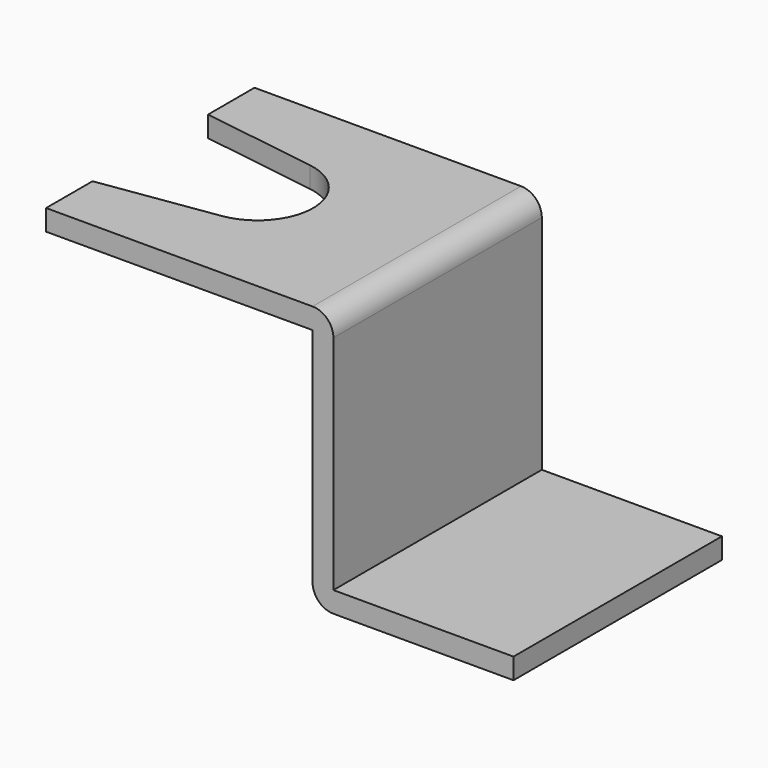
from build123d import *

# Parameters (mm, degrees)
F1_DEPTH = 25
F2_R     = 5.3407247833
F3_DEPTH = 25.3101193046
F5_DEPTH = 106
F6_DEPTH = 25.3101193046


# Not quite as in the source:
# - an extrude ends at something that could not be found from the text; its depth is read off the source's solid


with BuildPart() as f1:
    # F0 (on Front) → F1 (new body)
    with BuildSketch(Plane.XZ):
        with BuildLine():
            Line((-2, 0), (-58.1267029047, 0))
            Line((-58.1267029047, 0), (-58.1267029047, -2))
            Line((-58.1267029047, -2), (-2, -2))
            Line((-2, -2), (-2, -23.3091193046))
            ThreePointArc((-2, -23.3091193046), (-1.4142135624, -24.723332867), (0, -25.3091193046))
            Line((0, -25.3091193046), (17.2828252222, -25.3091193046))
            Line((17.2828252222, -25.3091193046), (17.2828252222, -23.3091193046))
            Line((17.2828252222, -23.3091193046), (0, -23.3091193046))
            Line((0, -23.3091193046), (0, -2))
            ThreePointArc((0, -2), (-0.5857864376, -0.5857864376), (-2, 0))
        make_face()
    extrude(amount=F1_DEPTH)

    # F2 (on face) → F3 (cut, through all)
    with BuildSketch(Plane.XY):
        with Locations((-17.279623447, -12.5)):
            Circle(F2_R)
    extrude(amount=-F3_DEPTH, mode=Mode.SUBTRACT)

    # F4 (on face) → F5 (cut, through all)
    with BuildSketch(Plane.XY):
        with BuildLine():
            Line((-27.5714416057, -5.5710808575), (-27.5714416057, 0))
            Line((-27.5714416057, 0), (-58.1267029047, 0))
            Line((-58.1267029047, 0), (-58.1267029047, -25))
            Line((-58.1267029047, -25), (-27.5714416057, -25))
            Line((-27.5714416057, -25), (-27.5714416057, -19.4289191425))
            Line((-27.5714416057, -19.4289191425), (-16.4945252417, -17.7827040443))
            ThreePointArc((-16.4945252417, -17.7827040443), (-22.6203482303, -12.5), (-16.4945252417, -7.2172959557))
            Line((-16.4945252417, -7.2172959557), (-27.5714416057, -5.5710808575))
        make_face()
    extrude(amount=F5_DEPTH, mode=Mode.SUBTRACT)

    # F4 (on face) → F6 (cut, through all)
    with BuildSketch(Plane.XY):
        with BuildLine():
            Line((-27.5714416057, -5.5710808575), (-27.5714416057, 0))
            Line((-27.5714416057, 0), (-58.1267029047, 0))
            Line((-58.1267029047, 0), (-58.1267029047, -25))
            Line((-58.1267029047, -25), (-27.5714416057, -25))
            Line((-27.5714416057, -25), (-27.5714416057, -19.4289191425))
            Line((-27.5714416057, -19.4289191425), (-16.4945252417, -17.7827040443))
            ThreePointArc((-16.4945252417, -17.7827040443), (-22.6203482303, -12.5), (-16.4945252417, -7.2172959557))
            Line((-16.4945252417, -7.2172959557), (-27.5714416057, -5.5710808575))
        make_face()
    extrude(amount=-F6_DEPTH, mode=Mode.SUBTRACT)


solid = f1.part
